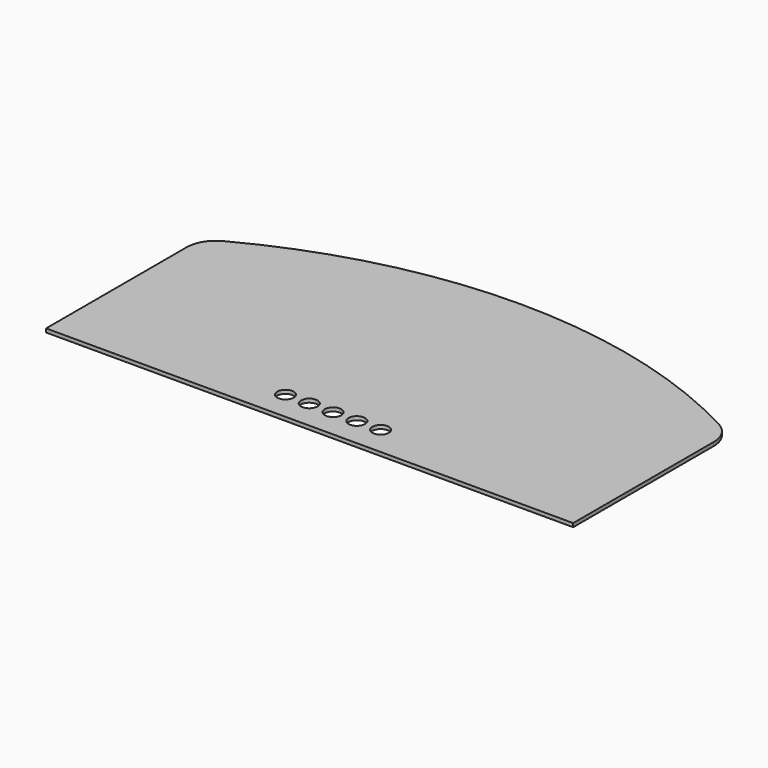
from build123d import *

# Parameters (mm, degrees)
F1_DEPTH = 6.35
F3_D     = 28.575


# Not quite as in the source:
# - a feature names something its author has since deleted; it is built from what else it names


with BuildPart() as f1:
    # F0 (on Top) → F1 (new body)
    with BuildSketch(Plane.XY):
        with BuildLine():
            Line((-914.4, 0), (0, 0))
            Line((0, 0), (0, 304.8))
            ThreePointArc((0, 304.8), (-7.2393593738, 330.9363843757), (-26.8941176471, 349.6235294118))
            ThreePointArc((-26.8941176471, 349.6235294118), (-457.2, 457.2), (-887.5058823529, 349.6235294118))
            ThreePointArc((-887.5058823529, 349.6235294118), (-907.1606406262, 330.9363843757), (-914.4, 304.8))
            Line((-914.4, 304.8), (-914.4, 0))
        make_face()
    extrude(amount=F1_DEPTH)

    # F3 (through all)
    with Locations(Plane(origin=(0, 0, 0), x_dir=(1, 0, 0), z_dir=(0, 0, -1))):
        with Locations((-415.925, -50.8), (-374.65, -50.8), (-457.2, -50.8), (-498.475, -50.8), (-539.75, -50.8)):
            Hole(F3_D / 2)


solid = f1.part
